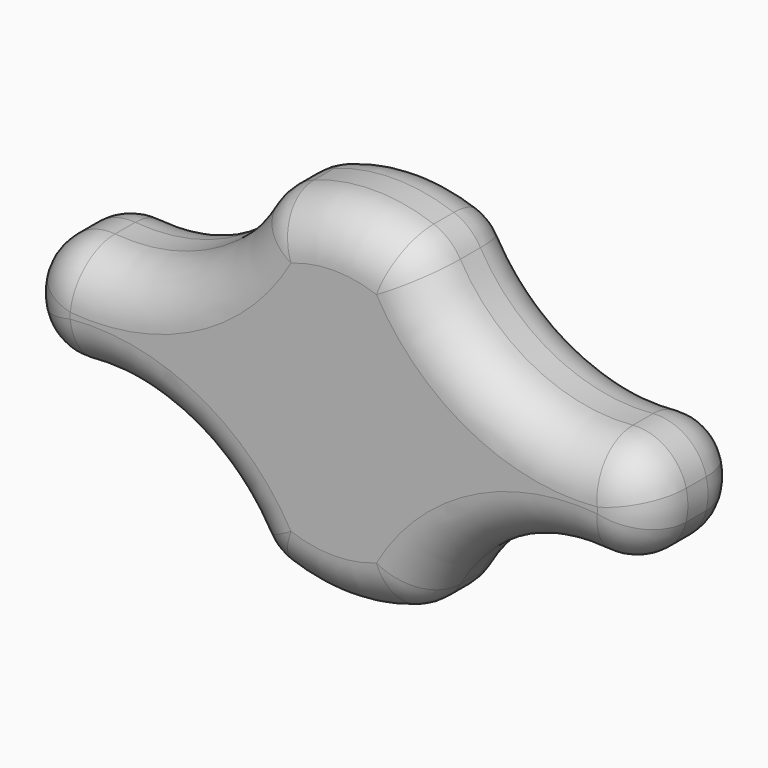
from build123d import *

# Parameters (mm, degrees)
F0_R     = 1
F1_DEPTH = 1
F2_R     = 3
F4_DEPTH = 1
F3_R     = 1
F5_DEPTH = 4
F7_DEPTH = 2.5
F8_R     = 2
F9_R     = 1


# Not quite as in the source:
# - the dataset's text gives a spline's control points without its knots; the knots are read off the source's solid


with BuildPart() as f1:
    # F0 (on Front) → F1 (new body, symmetric)
    with BuildSketch(Plane.XZ):
        with BuildLine():
            ThreePointArc((2.9469837534, -0.5615040135), (2.9867165299, -0.2820006559), (3, 0))
            ThreePointArc((3, 0), (2.9886065541, 0.2612103844), (2.9545127567, 0.5204367111))
            ThreePointArc((2.9545127567, 0.5204367111), (0.0271110209, 2.9998774963), (-2.9446241852, 0.5737494298))
            ThreePointArc((-2.9446241852, 0.5737494298), (-2.9998394671, 0.0310350097), (-2.9558641673, -0.5127055922))
            ThreePointArc((-2.9558641673, -0.5127055922), (-0.0247999379, -2.9998974921), (2.9469837534, -0.5615040135))
        make_face()
        Circle(F0_R, mode=Mode.SUBTRACT)
        with BuildLine():
            ThreePointArc((2.9545127567, 0.5204367111), (2.9886065541, 0.2612103844), (3, 0))
            ThreePointArc((3, 0), (2.9867165299, -0.2820006559), (2.9469837534, -0.5615040135))
            Line((2.9469837534, -0.5615040135), (3.2715276845, -0.4305277873))
            add(Edge.make_bspline(
                [(3.2715276845, -0.4305277873), (3.5872243405, -0.3031220567), (4.1559556498, 0.001609591), (4.7527348197, 0.6008364051), (5.0421686524, 1.3484439996), (5.0079249647, 2.0968992338), (4.7549524135, 2.7760434667), (4.3632157233, 3.3841015151), (3.8681556959, 3.9275260227), (3.0932594755, 4.5611414289), (2.1831247349, 5.0483299413), (1.2010595463, 5.3581588578), (0.4440987805, 5.4920848301), (-0.3198544585, 5.5135205052), (-1.3071208834, 5.3874592441), (-2.4607137336, 4.977077994), (-3.4536841153, 4.3070636741), (-4.1264235671, 3.6552364321), (-4.5573661081, 3.1197660917), (-4.9201984343, 2.5711055911), (-5.3500092381, 1.8417859277), (-5.7422540919, 1.1492953246), (-6.1699393691, 0.5525801025), (-6.5258390721, 0.160543319), (-6.9212446186, -0.1552690412), (-7.3435905834, -0.3640064182), (-7.7963916258, -0.4531389079), (-8.2005796684, -0.4145404292), (-8.4632307509, -0.334874547), (-8.5324493497, -0.3103144999)],
                knots=[0.0027902333, 0.0027902333, 0.0027902333, 0.0027902333, 0.03125, 0.0625, 0.09375, 0.125, 0.15625, 0.1875, 0.21875, 0.25, 0.3125, 0.34375, 0.375, 0.40625, 0.4375, 0.5, 0.5625, 0.59375, 0.625, 0.65625, 0.6875, 0.75, 0.78125, 0.8125, 0.84375, 0.875, 0.90625, 0.9375, 0.9482330782, 0.9482330782, 0.9482330782, 0.9482330782], degree=3))
            ThreePointArc((-8.5324493497, -0.3103144999), (-8.7241890465, -0.7888640003), (-9.0666296514, -1.1742315753))
            add(Edge.make_bspline(
                [(2.9545127567, 0.5204367111), (3.1827549994, 0.61670697), (3.5825117276, 0.8407033814), (3.9029540849, 1.1828573138), (4.0247487395, 1.5076386628), (4.0167623883, 1.8769581011), (3.8613731684, 2.3134171429), (3.5707234698, 2.7685743913), (3.1817273271, 3.1967475648), (2.5490925195, 3.7153477743), (1.5916945964, 4.2290472515), (0.5412107147, 4.4888935129), (-0.2678150291, 4.5111447002), (-1.0585479808, 4.4107036883), (-1.8124490087, 4.1437858665), (-2.4972171106, 3.7428060707), (-2.967429039, 3.3844249575), (-3.3852437142, 2.9794393308), (-3.8629554701, 2.3869367406), (-4.3739454298, 1.5361169449), (-4.884953201, 0.6291870777), (-5.3841894723, -0.0703753799), (-5.830213077, -0.5640752682), (-6.3678293325, -0.9974267167), (-7.0086442351, -1.3195310521), (-7.7532753579, -1.4675282847), (-8.4556923011, -1.3950863063), (-8.9012725561, -1.2442696683), (-9.0666296514, -1.1742315753)],
                knots=[0.0049249591, 0.0049249591, 0.0049249591, 0.0049249591, 0.03125, 0.0625, 0.09375, 0.125, 0.15625, 0.1875, 0.21875, 0.25, 0.3125, 0.375, 0.40625, 0.4375, 0.5, 0.53125, 0.5625, 0.59375, 0.625, 0.6875, 0.75, 0.78125, 0.8125, 0.84375, 0.875, 0.90625, 0.9375, 0.9555971311, 0.9555971311, 0.9555971311, 0.9555971311], degree=3))
        make_face()
        with BuildLine():
            ThreePointArc((-2.9558641673, -0.5127055922), (-2.9998394671, 0.0310350097), (-2.9446241852, 0.5737494298))
            Line((-2.9446241852, 0.5737494298), (-3.4130293264, 0.3826204136))
            add(Edge.make_bspline(
                [(-3.4130293264, 0.3826204136), (-3.6190534786, 0.2985538864), (-4.0683779313, 0.053395561), (-4.5889383513, -0.4876366395), (-4.8842626753, -1.2103729492), (-4.9222779191, -1.9621131384), (-4.7544951591, -2.6904992559), (-4.3008645586, -3.5898188832), (-3.3956432769, -4.4897516587), (-1.9970452848, -5.2141793244), (-0.7072103107, -5.5053880995), (0.3233385774, -5.5209585951), (1.3155419091, -5.3877503487), (2.4656367676, -4.9761029684), (3.4495042367, -4.3113809621), (4.1166146204, -3.6674463892), (4.546351148, -3.1392641684), (4.9108244184, -2.5973940215), (5.3452468336, -1.8756091097), (5.7443078845, -1.1864724201), (6.1794462863, -0.5854821097), (6.5415057068, -0.1855331004), (6.9424093073, 0.1405742205), (7.3682806356, 0.3584710003), (7.8191102446, 0.4537844509), (8.2143003633, 0.4194198664), (8.4695351569, 0.3429740418), (8.534567659, 0.3201687899)],
                knots=[0.0091008666, 0.0091008666, 0.0091008666, 0.0091008666, 0.03125, 0.0625, 0.09375, 0.125, 0.15625, 0.1875, 0.25, 0.3125, 0.375, 0.40625, 0.4375, 0.5, 0.5625, 0.59375, 0.625, 0.65625, 0.6875, 0.75, 0.78125, 0.8125, 0.84375, 0.875, 0.90625, 0.9375, 0.9477754589, 0.9477754589, 0.9477754589, 0.9477754589], degree=3))
            ThreePointArc((8.534567659, 0.3201687899), (8.7301439037, 0.7984143627), (9.0763921835, 1.181925802))
            add(Edge.make_bspline(
                [(-2.9558641673, -0.5127055922), (-3.1312941981, -0.5765718077), (-3.4443784148, -0.7438687766), (-3.7318457813, -1.0501521677), (-3.8872462828, -1.4242286977), (-3.9144072552, -1.8639366353), (-3.806121625, -2.3439754059), (-3.5725015597, -2.8112387766), (-3.2229929857, -3.2425596936), (-2.6184837876, -3.7607912269), (-1.6543098749, -4.263974376), (-0.3513972339, -4.5564595473), (0.8775185413, -4.4795676955), (1.818152778, -4.1430337834), (2.497543784, -3.7448112863), (2.9635134388, -3.3898454015), (3.3788444277, -2.9888521766), (3.8571053215, -2.4021004341), (4.3734486132, -1.5595331891), (4.9960868557, -0.4796058671), (5.6643087591, 0.3882087674), (6.3800905125, 0.9760640502), (7.0188946721, 1.3086851181), (7.7635093849, 1.4686410822), (8.4671627761, 1.4022164325), (8.9119960015, 1.2519419232), (9.0763921835, 1.181925802)],
                knots=[0.0050478584, 0.0050478584, 0.0050478584, 0.0050478584, 0.03125, 0.0625, 0.09375, 0.125, 0.15625, 0.1875, 0.21875, 0.25, 0.3125, 0.375, 0.4375, 0.5, 0.53125, 0.5625, 0.59375, 0.625, 0.6875, 0.75, 0.8125, 0.84375, 0.875, 0.90625, 0.9375, 0.955520936, 0.955520936, 0.955520936, 0.955520936], degree=3))
        make_face()
        with BuildLine():
            ThreePointArc((-8.5, 0), (-11.3509358835, 0.6518989481), (-9.0666296514, -1.1742315753))
            ThreePointArc((-9.0666296514, -1.1742315753), (-8.7241890465, -0.7888640003), (-8.5324493497, -0.3103144999))
            ThreePointArc((-8.5324493497, -0.3103144999), (-8.5081343936, -0.1560032445), (-8.5, 0))
        make_face()
        with Locations((-10, 0)):
            Circle(F0_R, mode=Mode.SUBTRACT)
        with BuildLine():
            ThreePointArc((11.5, 0), (10.657490789, 1.3482232242), (9.0763921835, 1.181925802))
            ThreePointArc((9.0763921835, 1.181925802), (8.7301439037, 0.7984143627), (8.534567659, 0.3201687899))
            ThreePointArc((8.534567659, 0.3201687899), (9.8389852669, -1.4913330465), (11.5, 0))
        make_face()
        with Locations((10, 0)):
            Circle(F0_R, mode=Mode.SUBTRACT)
    extrude(amount=F1_DEPTH, both=True)


with BuildPart() as f4:
    # F2 (on face) → F4 (new body)
    with BuildSketch(Plane(origin=(0, 1, 0), x_dir=(-1, 0, 0), z_dir=(0, 1, 0))):
        Circle(F2_R)
    extrude(amount=F4_DEPTH)


with BuildPart() as f5:
    # F3 (on Front) → F5 (new body)
    with BuildSketch(Plane.XZ):
        Circle(F3_R)
    extrude(amount=-F5_DEPTH)

    # F9
    f9_edges = [f5.edges().sort_by_distance(p)[0] for p in [
        (-1, 4, 0),
    ]]
    fillet(f9_edges, radius=F9_R)


with BuildPart() as f7:
    # F6 (on Front) → F7 (new body, symmetric)
    with BuildSketch(Plane.XZ):
        with BuildLine():
            ThreePointArc((10.3056206995, -2.110397389), (11.64886138, -1.7455376268), (12.4287431124, -0.592627112))
            ThreePointArc((12.4287431124, -0.592627112), (12.5, 0), (12.4287431124, 0.592627112))
            ThreePointArc((12.4287431124, 0.592627112), (11.64886138, 1.7455376268), (10.3056206995, 2.110397389))
            ThreePointArc((10.3056206995, 2.110397389), (6.3451749176, 2.8940155492), (3.4366713842, 5.6939790149))
            ThreePointArc((3.4366713842, 5.6939790149), (2.987453151, 6.2326030969), (2.3798971749, 6.5830152238))
            ThreePointArc((2.3798971749, 6.5830152238), (0, 7), (-2.3798971749, 6.5830152238))
            ThreePointArc((-2.3798971749, 6.5830152238), (-2.987453151, 6.2326030969), (-3.4366713842, 5.6939790149))
            ThreePointArc((-3.4366713842, 5.6939790149), (-6.3451749176, 2.8940155492), (-10.3056206995, 2.110397389))
            ThreePointArc((-10.3056206995, 2.110397389), (-11.64886138, 1.7455376268), (-12.4287431124, 0.592627112))
            ThreePointArc((-12.4287431124, 0.592627112), (-12.5, 0), (-12.4287431124, -0.592627112))
            ThreePointArc((-12.4287431124, -0.592627112), (-11.64886138, -1.7455376268), (-10.3056206995, -2.110397389))
            ThreePointArc((-10.3056206995, -2.110397389), (-6.3451749176, -2.8940155492), (-3.4366713842, -5.6939790149))
            ThreePointArc((-3.4366713842, -5.6939790149), (-2.987453151, -6.2326030969), (-2.3798971749, -6.5830152238))
            ThreePointArc((-2.3798971749, -6.5830152238), (0, -7), (2.3798971749, -6.5830152238))
            ThreePointArc((2.3798971749, -6.5830152238), (2.987453151, -6.2326030969), (3.4366713842, -5.6939790149))
            ThreePointArc((3.4366713842, -5.6939790149), (6.3451749176, -2.8940155492), (10.3056206995, -2.110397389))
        make_face()
    extrude(amount=F7_DEPTH, both=True)

    # F8
    f8_edges = [f7.edges().sort_by_distance(p)[0] for p in [
        (-6.345175, -2.5, 2.894016),
        (-6.345175, 2.5, -2.894016),
        (6.345175, 2.5, -2.894016),
        (6.345175, -2.5, -2.894016),
        (2.987453, 2.5, -6.232603),
        (2.987453, -2.5, -6.232603),
        (0, 2.5, -7),
        (0, -2.5, -7),
        (-2.987453, 2.5, -6.232603),
        (-2.987453, -2.5, -6.232603),
        (-6.345175, -2.5, -2.894016),
        (-11.648861, 2.5, -1.745538),
        (-11.648861, -2.5, -1.745538),
        (-12.5, 2.5, 0),
        (-12.5, -2.5, 0),
        (-11.648861, 2.5, 1.745538),
        (-11.648861, -2.5, 1.745538),
        (-6.345175, 2.5, 2.894016),
        (-2.987453, 2.5, 6.232603),
        (-2.987453, -2.5, 6.232603),
        (0, 2.5, 7),
        (0, -2.5, 7),
        (2.987453, 2.5, 6.232603),
        (2.987453, -2.5, 6.232603),
        (6.345175, 2.5, 2.894016),
        (6.345175, -2.5, 2.894016),
        (11.648861, 2.5, 1.745538),
        (11.648861, -2.5, 1.745538),
        (12.5, 2.5, 0),
        (12.5, -2.5, 0),
        (11.648861, -2.5, -1.745538),
        (11.648861, 2.5, -1.745538),
    ]]
    fillet(f8_edges, radius=F8_R)


solid = Compound([f1.part, f4.part, f5.part, f7.part])
